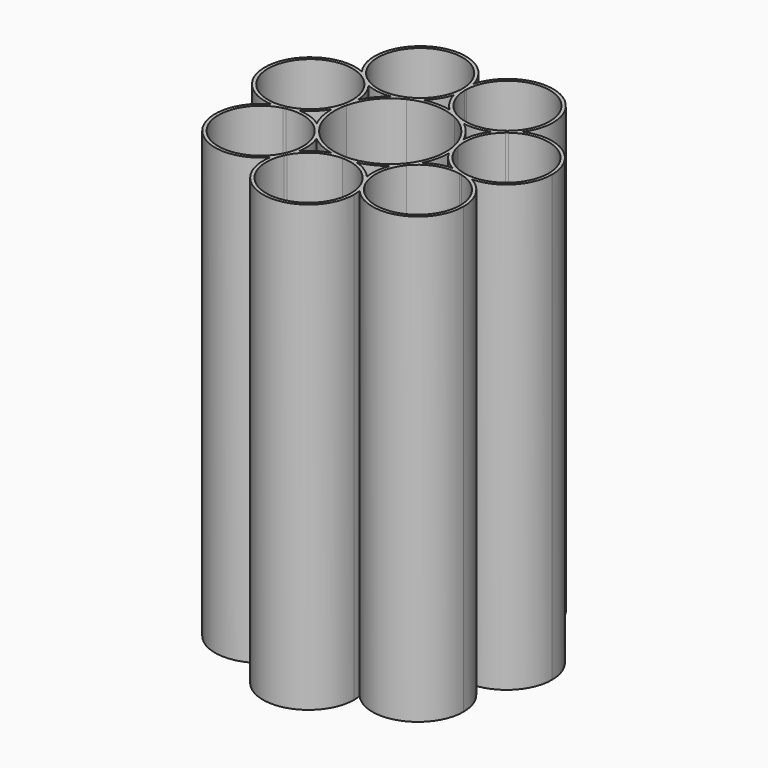
from build123d import *

# Parameters (mm, degrees)
F1_DEPTH = 100
F2_DEPTH = 1.5


with BuildPart() as f1:
    # F0 (on Top) → F1 (new body)
    with BuildSketch(Plane.XY):
        with BuildLine():
            ThreePointArc((48.1206952739, 11.3566633912), (48.7132972202, 9.4977687695), (48.9136480771, 7.5570148398))
            ThreePointArc((48.9136480771, 7.5570148398), (37.405752333, -1.7283690877), (30.7624155128, 11.4820849178))
            ThreePointArc((30.7624155128, 11.4820849178), (30.1118696666, 10.4093871837), (29.3351499151, 9.4241984938))
            ThreePointArc((29.3351499151, 9.4241984938), (38.476126387, -2.6500196502), (49.6636480771, 7.5570148398))
            ThreePointArc((49.6636480771, 7.5570148398), (49.6271899841, 8.4207634811), (49.5180750595, 9.2783676097))
            ThreePointArc((49.5180750595, 9.2783676097), (48.755672541, 10.2746771633), (48.1206952739, 11.3566633912))
        make_face()
        with BuildLine():
            ThreePointArc((47.8763467124, 11.8735796555), (48.0024107115, 11.6169602101), (48.1206952739, 11.3566633912))
            ThreePointArc((48.1206952739, 11.3566633912), (48.755672541, 10.2746771633), (49.5180750595, 9.2783676097))
            ThreePointArc((49.5180750595, 9.2783676097), (49.2321003695, 10.4998866655), (48.7990402105, 11.6773199866))
            ThreePointArc((48.7990402105, 11.6773199866), (48.6729762114, 11.933939432), (48.5546916491, 12.1942362509))
            ThreePointArc((48.5546916491, 12.1942362509), (47.919714382, 13.2762224787), (47.1573118635, 14.2725320324))
            ThreePointArc((47.1573118635, 14.2725320324), (47.4432865534, 13.0510129766), (47.8763467124, 11.8735796555))
        make_face()
        with BuildLine():
            ThreePointArc((29.3351499151, 9.4241984938), (30.1118696666, 10.4093871837), (30.7624155128, 11.4820849178))
            ThreePointArc((30.7624155128, 11.4820849178), (30.8844490564, 11.7406453283), (31.0142080859, 11.9954163351))
            ThreePointArc((31.0142080859, 11.9954163351), (31.464237132, 13.1664689319), (31.7678331121, 14.3837280695))
            ThreePointArc((31.7678331121, 14.3837280695), (30.9911133606, 13.3985393796), (30.3405675144, 12.3258416454))
            ThreePointArc((30.3405675144, 12.3258416454), (30.2185339708, 12.0672812349), (30.0887749413, 11.8125102282))
            ThreePointArc((30.0887749413, 11.8125102282), (29.6387458952, 10.6414576313), (29.3351499151, 9.4241984938))
        make_face()
        with BuildLine():
            ThreePointArc((39.4822879755, 17.0567668662), (44.4048695418, 15.6401892342), (47.8763467124, 11.8735796555))
            ThreePointArc((47.8763467124, 11.8735796555), (47.4432865534, 13.0510129766), (47.1573118635, 14.2725320324))
            ThreePointArc((47.1573118635, 14.2725320324), (44.9982610803, 16.1520481501), (42.4036526816, 17.3612166158))
            ThreePointArc((42.4036526816, 17.3612166158), (40.9514324879, 17.1277926143), (39.4822879755, 17.0567668662))
        make_face()
        with BuildLine():
            ThreePointArc((48.7990402105, 11.6773199866), (49.2321003695, 10.4998866655), (49.5180750595, 9.2783676097))
            ThreePointArc((49.5180750595, 9.2783676097), (60.8457272798, 6.3908890767), (67.5117388458, 15.9938848023))
            ThreePointArc((67.5117388458, 15.9938848023), (66.0890556448, 21.20358519), (62.215938235, 24.9670898268))
            ThreePointArc((62.215938235, 24.9670898268), (60.9616418645, 24.9922083817), (59.7198091175, 25.1703705424))
            ThreePointArc((59.7198091175, 25.1703705424), (64.7983716344, 21.7774102159), (66.7617388458, 15.9938848023))
            ThreePointArc((66.7617388458, 15.9938848023), (59.4814643879, 6.7568496439), (48.7990402105, 11.6773199866))
        make_face()
        with BuildLine():
            ThreePointArc((31.7678331121, 14.3837280695), (31.464237132, 13.1664689319), (31.0142080859, 11.9954163351))
            ThreePointArc((31.0142080859, 11.9954163351), (34.5397507817, 15.7114691534), (39.4822879755, 17.0567668662))
            ThreePointArc((39.4822879755, 17.0567668662), (38.0143233536, 17.149014592), (36.5656279622, 17.40339902))
            ThreePointArc((36.5656279622, 17.40339902), (33.9538177836, 16.2318493146), (31.7678331121, 14.3837280695))
        make_face()
        with BuildLine():
            ThreePointArc((16.8653170922, 25.294768849), (13.6295963948, 9.9182097392), (29.3351499151, 9.4241984938))
            ThreePointArc((29.3351499151, 9.4241984938), (29.6387458952, 10.6414576313), (30.0887749413, 11.8125102282))
            ThreePointArc((30.0887749413, 11.8125102282), (14.2193333623, 10.3815781771), (19.3641230306, 25.4619588697))
            ThreePointArc((19.3641230306, 25.4619588697), (18.1198454701, 25.3017599953), (16.8653170922, 25.294768849))
        make_face()
        with BuildLine():
            ThreePointArc((36.5656279622, 17.40339902), (38.0143233536, 17.149014592), (39.4822879755, 17.0567668662))
            ThreePointArc((39.4822879755, 17.0567668662), (40.9514324879, 17.1277926143), (42.4036526816, 17.3612166158))
            ThreePointArc((42.4036526816, 17.3612166158), (40.9617908418, 17.6894259043), (39.4877071959, 17.8067472874))
            ThreePointArc((39.4877071959, 17.8067472874), (38.0120820394, 17.7107389173), (36.5656279622, 17.40339902))
        make_face()
        with BuildLine():
            ThreePointArc((47.7878142081, 19.9063331353), (47.0753316403, 17.1338884178), (47.1573118635, 14.2725320324))
            ThreePointArc((47.1573118635, 14.2725320324), (47.919714382, 13.2762224787), (48.5546916491, 12.1942362509))
            ThreePointArc((48.5546916491, 12.1942362509), (47.8475044956, 17.2675376586), (49.8773300395, 21.9705483013))
            ThreePointArc((49.8773300395, 21.9705483013), (48.8899468368, 20.8803627751), (47.7878142081, 19.9063331353))
        make_face()
        with BuildLine():
            ThreePointArc((30.3405675144, 12.3258416454), (30.9911133606, 13.3985393796), (31.7678331121, 14.3837280695))
            ThreePointArc((31.7678331121, 14.3837280695), (31.8963694401, 15.3133900333), (31.9393349501, 16.2509117234))
            ThreePointArc((31.9393349501, 16.2509117234), (31.7575914431, 18.1725545596), (31.2188059374, 20.0260518137))
            ThreePointArc((31.2188059374, 20.0260518137), (30.1308632886, 21.0159057298), (29.1593365515, 22.1202452524))
            ThreePointArc((29.1593365515, 22.1202452524), (30.6675033383, 19.3561480096), (31.1893349501, 16.2509117234))
            ThreePointArc((31.1893349501, 16.2509117234), (30.9747188775, 14.2430159793), (30.3405675144, 12.3258416454))
        make_face()
        with BuildLine():
            ThreePointArc((19.2024519144, 26.1946490876), (18.0062976057, 25.8163566122), (16.8653170922, 25.294768849))
            ThreePointArc((16.8653170922, 25.294768849), (18.1198454701, 25.3017599953), (19.3641230306, 25.4619588697))
            ThreePointArc((19.3641230306, 25.4619588697), (19.6423603695, 25.5277589824), (19.922451795, 25.5851564126))
            ThreePointArc((19.922451795, 25.5851564126), (21.1186061037, 25.9634488879), (22.2595866172, 26.4850366512))
            ThreePointArc((22.2595866172, 26.4850366512), (21.0050582393, 26.4780455049), (19.7607806788, 26.3178466305))
            ThreePointArc((19.7607806788, 26.3178466305), (19.4825433399, 26.2520465177), (19.2024519144, 26.1946490876))
        make_face()
        with BuildLine():
            ThreePointArc((21.4986150447, 44.9392154972), (7.4592981841, 37.8818760143), (16.8653170922, 25.294768849))
            ThreePointArc((16.8653170922, 25.294768849), (18.0062976057, 25.8163566122), (19.2024519144, 26.1946490876))
            ThreePointArc((19.2024519144, 26.1946490876), (8.1892692018, 37.7097065822), (23.1873094858, 43.0898116188))
            ThreePointArc((23.1873094858, 43.0898116188), (22.2862665927, 43.9627446242), (21.4986150447, 44.9392154972))
        make_face()
        with BuildLine():
            ThreePointArc((31.2188059374, 20.0260518137), (33.7429593868, 18.4104328977), (36.5656279622, 17.40339902))
            ThreePointArc((36.5656279622, 17.40339902), (38.0120820394, 17.7107389173), (39.4877071959, 17.8067472874))
            ThreePointArc((39.4877071959, 17.8067472874), (34.0732460725, 19.0837906816), (29.7490735348, 22.5836136702))
            ThreePointArc((29.7490735348, 22.5836136702), (30.5764241251, 21.3579799622), (31.2188059374, 20.0260518137))
        make_face()
        with BuildLine():
            ThreePointArc((39.4877071959, 17.8067472874), (40.9617908418, 17.6894259043), (42.4036526816, 17.3612166158))
            ThreePointArc((42.4036526816, 17.3612166158), (45.2405783478, 18.3273573313), (47.7878142081, 19.9063331353))
            ThreePointArc((47.7878142081, 19.9063331353), (48.4493754616, 21.2288395857), (49.2943501781, 22.4423898862))
            ThreePointArc((49.2943501781, 22.4423898862), (44.9200562534, 19.005417496), (39.4877071959, 17.8067472874))
        make_face()
        with BuildLine():
            ThreePointArc((49.2943501781, 22.4423898862), (48.4493754616, 21.2288395857), (47.7878142081, 19.9063331353))
            ThreePointArc((47.7878142081, 19.9063331353), (48.8899468368, 20.8803627751), (49.8773300395, 21.9705483013))
            ThreePointArc((49.8773300395, 21.9705483013), (50.737796422, 23.1634554911), (51.4607426152, 24.4443843575))
            ThreePointArc((51.4607426152, 24.4443843575), (50.3051519569, 23.5217263825), (49.2943501781, 22.4423898862))
        make_face()
        with BuildLine():
            ThreePointArc((59.7198091175, 25.1703705424), (60.9616418645, 24.9922083817), (62.215938235, 24.9670898268))
            ThreePointArc((62.215938235, 24.9670898268), (61.082613878, 25.505110485), (59.8920508463, 25.900648087))
            ThreePointArc((59.8920508463, 25.900648087), (59.612818067, 25.9620868909), (59.3355606009, 26.0319007082))
            ThreePointArc((59.3355606009, 26.0319007082), (58.0937278539, 26.210062869), (56.8394314834, 26.2351814239))
            ThreePointArc((56.8394314834, 26.2351814239), (57.9727558404, 25.6971607656), (59.1633188721, 25.3016231636))
            ThreePointArc((59.1633188721, 25.3016231636), (59.4425516513, 25.2401843598), (59.7198091175, 25.1703705424))
        make_face()
        with BuildLine():
            ThreePointArc((59.8920508463, 25.900648087), (61.082613878, 25.505110485), (62.215938235, 24.9670898268))
            ThreePointArc((62.215938235, 24.9670898268), (69.1892765667, 28.1114205638), (72.0436308726, 35.2083864484))
            ThreePointArc((72.0436308726, 35.2083864484), (67.4863642116, 43.732193528), (57.8669894813, 44.6764373241))
            ThreePointArc((57.8669894813, 44.6764373241), (57.0653100087, 43.711450096), (56.1517471691, 42.8516284488))
            ThreePointArc((56.1517471691, 42.8516284488), (66.0745247522, 43.6891852074), (71.2936308726, 35.2083864484))
            ThreePointArc((71.2936308726, 35.2083864484), (67.8013338342, 27.849208157), (59.8920508463, 25.900648087))
        make_face()
        with BuildLine():
            ThreePointArc((23.6593494729, 43.6730360661), (22.6177984932, 44.372365662), (21.4986150447, 44.9392154972))
            ThreePointArc((21.4986150447, 44.9392154972), (22.2862665927, 43.9627446242), (23.1873094858, 43.0898116188))
            ThreePointArc((23.1873094858, 43.0898116188), (23.4122322289, 42.913302607), (23.6317414941, 42.7301050249))
            ThreePointArc((23.6317414941, 42.7301050249), (24.6732924738, 42.030775429), (25.7924759223, 41.4639255938))
            ThreePointArc((25.7924759223, 41.4639255938), (25.0048243743, 42.4403964668), (24.1037814812, 43.3133294722))
            ThreePointArc((24.1037814812, 43.3133294722), (23.8788587381, 43.489838484), (23.6593494729, 43.6730360661))
        make_face()
        with BuildLine():
            ThreePointArc((39.7460759123, 53.5648694386), (25.4750548344, 60.1410701567), (21.4986150447, 44.9392154972))
            ThreePointArc((21.4986150447, 44.9392154972), (22.6177984932, 44.372365662), (23.6593494729, 43.6730360661))
            ThreePointArc((23.6593494729, 43.6730360661), (25.7955768373, 59.4630099487), (39.3530374989, 51.0915105026))
            ThreePointArc((39.3530374989, 51.0915105026), (39.4737329496, 52.34023903), (39.7460759123, 53.5648694386))
        make_face()
        with BuildLine():
            ThreePointArc((29.1593365515, 22.1202452524), (30.1308632886, 21.0159057298), (31.2188059374, 20.0260518137))
            ThreePointArc((31.2188059374, 20.0260518137), (30.5764241251, 21.3579799622), (29.7490735348, 22.5836136702))
            ThreePointArc((29.7490735348, 22.5836136702), (28.7539739464, 23.6774436092), (27.6118365935, 24.6167036336))
            ThreePointArc((27.6118365935, 24.6167036336), (28.3161976905, 23.3254617924), (29.1593365515, 22.1202452524))
        make_face()
        with BuildLine():
            ThreePointArc((51.4607426152, 24.4443843575), (50.737796422, 23.1634554911), (49.8773300395, 21.9705483013))
            ThreePointArc((49.8773300395, 21.9705483013), (54.054034403, 24.935955715), (59.1633188721, 25.3016231636))
            ThreePointArc((59.1633188721, 25.3016231636), (57.9727558404, 25.6971607656), (56.8394314834, 26.2351814239))
            ThreePointArc((56.8394314834, 26.2351814239), (54.0238204657, 25.7190266811), (51.4607426152, 24.4443843575))
        make_face()
        with BuildLine():
            ThreePointArc((52.0780229629, 30.3064210056), (51.3615727292, 26.1353354269), (49.2943501781, 22.4423898862))
            ThreePointArc((49.2943501781, 22.4423898862), (50.3051519569, 23.5217263825), (51.4607426152, 24.4443843575))
            ThreePointArc((51.4607426152, 24.4443843575), (52.4741776089, 27.26476104), (52.8278601971, 30.24074554))
            ThreePointArc((52.8278601971, 30.24074554), (52.2063596702, 31.5825443542), (51.7844009488, 32.9998085498))
            ThreePointArc((51.7844009488, 32.9998085498), (52.0044006496, 31.6610935076), (52.0780229629, 30.3064210056))
        make_face()
        with BuildLine():
            ThreePointArc((22.2595866172, 26.4850366512), (21.1186061037, 25.9634488879), (19.922451795, 25.5851564126))
            ThreePointArc((19.922451795, 25.5851564126), (25.0259188828, 25.145697143), (29.1593365515, 22.1202452524))
            ThreePointArc((29.1593365515, 22.1202452524), (28.3161976905, 23.3254617924), (27.6118365935, 24.6167036336))
            ThreePointArc((27.6118365935, 24.6167036336), (25.0674451398, 25.9282497637), (22.2595866172, 26.4850366512))
        make_face()
        with BuildLine():
            ThreePointArc((40.1033328511, 51.0860892748), (40.0006943318, 52.3364314925), (39.7460759123, 53.5648694386))
            ThreePointArc((39.7460759123, 53.5648694386), (39.4737329496, 52.34023903), (39.3530374989, 51.0915105026))
            ThreePointArc((39.3530374989, 51.0915105026), (39.3549010101, 50.9828860122), (39.3555222076, 50.8742473143))
            ThreePointArc((39.3555222076, 50.8742473143), (39.3538681077, 50.6969758782), (39.3489063841, 50.5197661737))
            ThreePointArc((39.3489063841, 50.5197661737), (39.4515449033, 49.269423956), (39.7061633229, 48.0409860099))
            ThreePointArc((39.7061633229, 48.0409860099), (39.9785062855, 49.2656164185), (40.0992017363, 50.5143449459))
            ThreePointArc((40.0992017363, 50.5143449459), (40.0969650022, 50.8002481964), (40.1033328511, 51.0860892748))
        make_face()
        with BuildLine():
            ThreePointArc((59.8467170275, 50.7316081342), (51.0273512521, 60.8812773759), (39.7460759123, 53.5648694386))
            ThreePointArc((39.7460759123, 53.5648694386), (40.0006943318, 52.3364314925), (40.1033328511, 51.0860892748))
            ThreePointArc((40.1033328511, 51.0860892748), (49.7739884636, 60.2299540343), (59.0967170275, 50.7316081342))
            ThreePointArc((59.0967170275, 50.7316081342), (58.2024981574, 46.7078622248), (55.6881841552, 43.4416130565))
            ThreePointArc((55.6881841552, 43.4416130565), (56.7397318136, 44.1258190555), (57.8669894813, 44.6764373241))
            ThreePointArc((57.8669894813, 44.6764373241), (59.3392216503, 47.5463132225), (59.8467170275, 50.7316081342))
        make_face()
        with BuildLine():
            ThreePointArc((26.68186832, 33.3480809845), (24.2054297809, 28.8641370859), (19.7607806788, 26.3178466305))
            ThreePointArc((19.7607806788, 26.3178466305), (21.0050582393, 26.4780455049), (22.2595866172, 26.4850366512))
            ThreePointArc((22.2595866172, 26.4850366512), (24.5724133385, 28.1717238416), (26.3286201104, 30.4322146944))
            ThreePointArc((26.3286201104, 30.4322146944), (26.4241979206, 31.8999663481), (26.68186832, 33.3480809845))
        make_face()
        with BuildLine():
            ThreePointArc((27.6118365935, 24.6167036336), (28.7539739464, 23.6774436092), (29.7490735348, 22.5836136702))
            ThreePointArc((29.7490735348, 22.5836136702), (27.3716449829, 27.613033434), (27.4118393617, 33.1759116542))
            ThreePointArc((27.4118393617, 33.1759116542), (26.9694449908, 31.7648927136), (26.3286201104, 30.4322146944))
            ThreePointArc((26.3286201104, 30.4322146944), (26.6392623122, 27.4514301433), (27.6118365935, 24.6167036336))
        make_face()
        with BuildLine():
            ThreePointArc((56.8394314834, 26.2351814239), (58.0937278539, 26.210062869), (59.3355606009, 26.0319007082))
            ThreePointArc((59.3355606009, 26.0319007082), (54.9281698401, 28.64215124), (52.5167835917, 33.1614119671))
            ThreePointArc((52.5167835917, 33.1614119671), (52.7499833016, 31.7423739415), (52.8280229629, 30.3064210056))
            ThreePointArc((52.8280229629, 30.3064210056), (52.8279822714, 30.2735831719), (52.8278601971, 30.24074554))
            ThreePointArc((52.8278601971, 30.24074554), (54.5512191456, 27.9551132302), (56.8394314834, 26.2351814239))
        make_face()
        with BuildLine():
            ThreePointArc((56.1517471691, 42.8516284488), (57.0653100087, 43.711450096), (57.8669894813, 44.6764373241))
            ThreePointArc((57.8669894813, 44.6764373241), (56.7397318136, 44.1258190555), (55.6881841552, 43.4416130565))
            ThreePointArc((55.6881841552, 43.4416130565), (55.4660505739, 43.2616065464), (55.238600731, 43.0883661338))
            ThreePointArc((55.238600731, 43.0883661338), (54.3250378913, 42.2285444866), (53.5233584188, 41.2635572585))
            ThreePointArc((53.5233584188, 41.2635572585), (54.6506160864, 41.8141755271), (55.7021637449, 42.4983815261))
            ThreePointArc((55.7021637449, 42.4983815261), (55.9242973262, 42.6783880362), (56.1517471691, 42.8516284488))
        make_face()
        with BuildLine():
            ThreePointArc((25.7924759223, 41.4639255938), (24.6732924738, 42.030775429), (23.6317414941, 42.7301050249))
            ThreePointArc((23.6317414941, 42.7301050249), (26.0701979054, 39.4903555662), (26.9355687593, 35.5288937767))
            ThreePointArc((26.9355687593, 35.5288937767), (26.8719305007, 34.4311337452), (26.68186832, 33.3480809845))
            ThreePointArc((26.68186832, 33.3480809845), (27.0984560706, 34.7587136939), (27.6688276266, 36.1144814773))
            ThreePointArc((27.6688276266, 36.1144814773), (27.1078335586, 38.9215024564), (25.7924759223, 41.4639255938))
        make_face()
        with BuildLine():
            ThreePointArc((33.9154678115, 42.2854847903), (28.8657450324, 41.4259489943), (24.1037814812, 43.3133294722))
            ThreePointArc((24.1037814812, 43.3133294722), (25.0048243743, 42.4403964668), (25.7924759223, 41.4639255938))
            ThreePointArc((25.7924759223, 41.4639255938), (28.5532049431, 40.7073171118), (31.4155048698, 40.7436523617))
            ThreePointArc((31.4155048698, 40.7436523617), (32.6226312153, 41.5840548726), (33.9154678115, 42.2854847903))
        make_face()
        with BuildLine():
            ThreePointArc((27.6688276266, 36.1144814773), (27.0984560706, 34.7587136939), (26.68186832, 33.3480809845))
            ThreePointArc((26.68186832, 33.3480809845), (26.4241979206, 31.8999663481), (26.3286201104, 30.4322146944))
            ThreePointArc((26.3286201104, 30.4322146944), (26.9694449908, 31.7648927136), (27.4118393617, 33.1759116542))
            ThreePointArc((27.4118393617, 33.1759116542), (27.6169064336, 34.3444685309), (27.6855687593, 35.5288937767))
            ThreePointArc((27.6855687593, 35.5288937767), (27.6813826214, 35.821807254), (27.6688276266, 36.1144814773))
        make_face()
        with BuildLine():
            ThreePointArc((27.6855687593, 35.5288937767), (27.6169064336, 34.3444685309), (27.4118393617, 33.1759116542))
            ThreePointArc((27.4118393617, 33.1759116542), (29.8616956216, 38.1704519693), (34.2359896665, 41.6074245124))
            ThreePointArc((34.2359896665, 41.6074245124), (32.8569822677, 41.0735464461), (31.4155048698, 40.7436523617))
            ThreePointArc((31.4155048698, 40.7436523617), (29.2787159102, 38.6422937394), (27.6688276266, 36.1144814773))
            ThreePointArc((27.6688276266, 36.1144814773), (27.6813826214, 35.821807254), (27.6855687593, 35.5288937767))
        make_face()
        with BuildLine():
            ThreePointArc((51.7844009488, 32.9998085498), (52.2063596702, 31.5825443542), (52.8278601971, 30.24074554))
            ThreePointArc((52.8278601971, 30.24074554), (52.8279822714, 30.2735831719), (52.8280229629, 30.3064210056))
            ThreePointArc((52.8280229629, 30.3064210056), (52.7499833016, 31.7423739415), (52.5167835917, 33.1614119671))
            ThreePointArc((52.5167835917, 33.1614119671), (52.1206232128, 34.5779171099), (51.5699022873, 35.9417852589))
            ThreePointArc((51.5699022873, 35.9417852589), (51.5707663403, 34.4630403849), (51.7844009488, 32.9998085498))
        make_face()
        with BuildLine():
            ThreePointArc((45.0828000959, 41.5290512105), (49.4069725, 38.0292282022), (51.7844009488, 32.9998085498))
            ThreePointArc((51.7844009488, 32.9998085498), (51.5707663403, 34.4630403849), (51.5699022873, 35.9417852589))
            ThreePointArc((51.5699022873, 35.9417852589), (49.9967093879, 38.4925967413), (47.8905085013, 40.6246129099))
            ThreePointArc((47.8905085013, 40.6246129099), (46.4539487673, 40.9753020883), (45.0828000959, 41.5290512105))
        make_face()
        with BuildLine():
            ThreePointArc((51.5699022873, 35.9417852589), (52.1206232128, 34.5779171099), (52.5167835917, 33.1614119671))
            ThreePointArc((52.5167835917, 33.1614119671), (52.8024673174, 38.2757921802), (55.7021637449, 42.4983815261))
            ThreePointArc((55.7021637449, 42.4983815261), (54.6506160864, 41.8141755271), (53.5233584188, 41.2635572585))
            ThreePointArc((53.5233584188, 41.2635572585), (52.171399691, 38.7404067043), (51.5699022873, 35.9417852589))
        make_face()
        with BuildLine():
            ThreePointArc((39.7061633229, 48.0409860099), (39.4515449033, 49.269423956), (39.3489063841, 50.5197661737))
            ThreePointArc((39.3489063841, 50.5197661737), (37.7848370903, 45.6420426651), (33.9154678115, 42.2854847903))
            ThreePointArc((33.9154678115, 42.2854847903), (35.2780829825, 42.8392984152), (36.6936856513, 43.238671323))
            ThreePointArc((36.6936856513, 43.238671323), (38.5385289443, 45.4274231009), (39.7061633229, 48.0409860099))
        make_face()
        with BuildLine():
            ThreePointArc((45.4130863949, 42.2024091841), (41.5926238575, 45.6145296195), (40.0992017363, 50.5143449459))
            ThreePointArc((40.0992017363, 50.5143449459), (39.9785062855, 49.2656164185), (39.7061633229, 48.0409860099))
            ThreePointArc((39.7061633229, 48.0409860099), (40.8359093819, 45.4108234744), (42.6489322384, 43.1956419371))
            ThreePointArc((42.6489322384, 43.1956419371), (44.0586161482, 42.7758550227), (45.4130863949, 42.2024091841))
        make_face()
        with BuildLine():
            ThreePointArc((36.6936856513, 43.238671323), (35.2780829825, 42.8392984152), (33.9154678115, 42.2854847903))
            ThreePointArc((33.9154678115, 42.2854847903), (32.6226312153, 41.5840548726), (31.4155048698, 40.7436523617))
            ThreePointArc((31.4155048698, 40.7436523617), (32.8569822677, 41.0735464461), (34.2359896665, 41.6074245124))
            ThreePointArc((34.2359896665, 41.6074245124), (35.5238254256, 42.3341747953), (36.6936856513, 43.238671323))
        make_face()
        with BuildLine():
            ThreePointArc((36.6936856513, 43.238671323), (35.5238254256, 42.3341747953), (34.2359896665, 41.6074245124))
            ThreePointArc((34.2359896665, 41.6074245124), (39.6683389786, 42.806094722), (45.0828000959, 41.5290512105))
            ThreePointArc((45.0828000959, 41.5290512105), (43.8056003177, 42.2743350954), (42.6489322384, 43.1956419371))
            ThreePointArc((42.6489322384, 43.1956419371), (39.6737577864, 43.5560751461), (36.6936856513, 43.238671323))
        make_face()
        with BuildLine():
            ThreePointArc((42.6489322384, 43.1956419371), (43.8056003177, 42.2743350954), (45.0828000959, 41.5290512105))
            ThreePointArc((45.0828000959, 41.5290512105), (46.4539487673, 40.9753020883), (47.8905085013, 40.6246129099))
            ThreePointArc((47.8905085013, 40.6246129099), (46.6956521847, 41.4823708203), (45.4130863949, 42.2024091841))
            ThreePointArc((45.4130863949, 42.2024091841), (44.0586161482, 42.7758550227), (42.6489322384, 43.1956419371))
        make_face()
        with BuildLine():
            ThreePointArc((53.5233584188, 41.2635572585), (54.3250378913, 42.2285444866), (55.238600731, 43.0883661338))
            ThreePointArc((55.238600731, 43.0883661338), (50.4498614665, 41.2699938657), (45.4130863949, 42.2024091841))
            ThreePointArc((45.4130863949, 42.2024091841), (46.6956521847, 41.4823708203), (47.8905085013, 40.6246129099))
            ThreePointArc((47.8905085013, 40.6246129099), (50.7519845278, 40.5469207555), (53.5233584188, 41.2635572585))
        make_face()
    extrude(amount=F1_DEPTH)

    # F0 (on Top) → F2 (join)
    with BuildSketch(Plane.XY):
        with BuildLine():
            ThreePointArc((30.7624155128, 11.4820849178), (37.405752333, -1.7283690877), (48.9136480771, 7.5570148398))
            ThreePointArc((48.9136480771, 7.5570148398), (48.7132972202, 9.4977687695), (48.1206952739, 11.3566633912))
            ThreePointArc((48.1206952739, 11.3566633912), (47.9949160034, 11.613417429), (47.8763467124, 11.8735796555))
            ThreePointArc((47.8763467124, 11.8735796555), (44.4048695418, 15.6401892342), (39.4822879755, 17.0567668662))
            ThreePointArc((39.4822879755, 17.0567668662), (34.5397507817, 15.7114691534), (31.0142080859, 11.9954163351))
            ThreePointArc((31.0142080859, 11.9954163351), (30.8918917882, 11.7369946174), (30.7624155128, 11.4820849178))
        make_face()
        with BuildLine():
            ThreePointArc((39.4822879755, 17.0567668662), (44.4048695418, 15.6401892342), (47.8763467124, 11.8735796555))
            ThreePointArc((47.8763467124, 11.8735796555), (47.4432865534, 13.0510129766), (47.1573118635, 14.2725320324))
            ThreePointArc((47.1573118635, 14.2725320324), (44.9982610803, 16.1520481501), (42.4036526816, 17.3612166158))
            ThreePointArc((42.4036526816, 17.3612166158), (40.9514324879, 17.1277926143), (39.4822879755, 17.0567668662))
        make_face()
        with BuildLine():
            ThreePointArc((48.5546916491, 12.1942362509), (48.6804709195, 11.937482213), (48.7990402105, 11.6773199866))
            ThreePointArc((48.7990402105, 11.6773199866), (59.4814643879, 6.7568496439), (66.7617388458, 15.9938848023))
            ThreePointArc((66.7617388458, 15.9938848023), (64.7983716344, 21.7774102159), (59.7198091175, 25.1703705424))
            ThreePointArc((59.7198091175, 25.1703705424), (59.440648635, 25.2321158732), (59.1633188721, 25.3016231636))
            ThreePointArc((59.1633188721, 25.3016231636), (54.054034403, 24.935955715), (49.8773300395, 21.9705483013))
            ThreePointArc((49.8773300395, 21.9705483013), (47.8475044956, 17.2675376586), (48.5546916491, 12.1942362509))
        make_face()
        with BuildLine():
            ThreePointArc((19.3641230306, 25.4619588697), (14.2193333623, 10.3815781771), (30.0887749413, 11.8125102282))
            ThreePointArc((30.0887749413, 11.8125102282), (30.211091239, 12.0709319458), (30.3405675144, 12.3258416454))
            ThreePointArc((30.3405675144, 12.3258416454), (30.9747188775, 14.2430159793), (31.1893349501, 16.2509117234))
            ThreePointArc((31.1893349501, 16.2509117234), (30.6675033383, 19.3561480096), (29.1593365515, 22.1202452524))
            ThreePointArc((29.1593365515, 22.1202452524), (25.0259188828, 25.145697143), (19.922451795, 25.5851564126))
            ThreePointArc((19.922451795, 25.5851564126), (19.6441465962, 25.5196638394), (19.3641230306, 25.4619588697))
        make_face()
        with BuildLine():
            ThreePointArc((23.1873094858, 43.0898116188), (8.1892692018, 37.7097065822), (19.2024519144, 26.1946490876))
            ThreePointArc((19.2024519144, 26.1946490876), (19.4807571132, 26.2601416608), (19.7607806788, 26.3178466305))
            ThreePointArc((19.7607806788, 26.3178466305), (24.2054297809, 28.8641370859), (26.68186832, 33.3480809845))
            ThreePointArc((26.68186832, 33.3480809845), (26.8719305007, 34.4311337452), (26.9355687593, 35.5288937767))
            ThreePointArc((26.9355687593, 35.5288937767), (26.0701979054, 39.4903555662), (23.6317414941, 42.7301050249))
            ThreePointArc((23.6317414941, 42.7301050249), (23.4070168853, 42.9068588395), (23.1873094858, 43.0898116188))
        make_face()
        with BuildLine():
            ThreePointArc((29.7490735348, 22.5836136702), (34.0732460725, 19.0837906816), (39.4877071959, 17.8067472874))
            ThreePointArc((39.4877071959, 17.8067472874), (44.9200562534, 19.005417496), (49.2943501781, 22.4423898862))
            ThreePointArc((49.2943501781, 22.4423898862), (51.3615727292, 26.1353354269), (52.0780229629, 30.3064210056))
            ThreePointArc((52.0780229629, 30.3064210056), (52.0044006496, 31.6610935076), (51.7844009488, 32.9998085498))
            ThreePointArc((51.7844009488, 32.9998085498), (49.4069725, 38.0292282022), (45.0828000959, 41.5290512105))
            ThreePointArc((45.0828000959, 41.5290512105), (39.6683389786, 42.806094722), (34.2359896665, 41.6074245124))
            ThreePointArc((34.2359896665, 41.6074245124), (29.8616956216, 38.1704519693), (27.4118393617, 33.1759116542))
            ThreePointArc((27.4118393617, 33.1759116542), (27.3716449829, 27.613033434), (29.7490735348, 22.5836136702))
        make_face()
        with BuildLine():
            ThreePointArc((59.3355606009, 26.0319007082), (59.6147210834, 25.9701553775), (59.8920508463, 25.900648087))
            ThreePointArc((59.8920508463, 25.900648087), (67.8013338342, 27.849208157), (71.2936308726, 35.2083864484))
            ThreePointArc((71.2936308726, 35.2083864484), (66.0745247522, 43.6891852074), (56.1517471691, 42.8516284488))
            ThreePointArc((56.1517471691, 42.8516284488), (55.9294190118, 42.671869579), (55.7021637449, 42.4983815261))
            ThreePointArc((55.7021637449, 42.4983815261), (52.8024673174, 38.2757921802), (52.5167835917, 33.1614119671))
            ThreePointArc((52.5167835917, 33.1614119671), (54.9281698401, 28.64215124), (59.3355606009, 26.0319007082))
        make_face()
        with BuildLine():
            ThreePointArc((39.3530374989, 51.0915105026), (25.7955768373, 59.4630099487), (23.6593494729, 43.6730360661))
            ThreePointArc((23.6593494729, 43.6730360661), (23.8840740817, 43.4962822514), (24.1037814812, 43.3133294722))
            ThreePointArc((24.1037814812, 43.3133294722), (28.8657450324, 41.4259489943), (33.9154678115, 42.2854847903))
            ThreePointArc((33.9154678115, 42.2854847903), (37.7848370903, 45.6420426651), (39.3489063841, 50.5197661737))
            ThreePointArc((39.3489063841, 50.5197661737), (39.3469845792, 50.8056671487), (39.3530374989, 51.0915105026))
        make_face()
        with BuildLine():
            ThreePointArc((59.0967170275, 50.7316081342), (49.7739884636, 60.2299540343), (40.1033328511, 51.0860892748))
            ThreePointArc((40.1033328511, 51.0860892748), (40.1049748539, 50.9801739511), (40.1055222076, 50.8742473143))
            ThreePointArc((40.1055222076, 50.8742473143), (40.103941968, 50.6942683828), (40.0992017363, 50.5143449459))
            ThreePointArc((40.0992017363, 50.5143449459), (41.5926238575, 45.6145296195), (45.4130863949, 42.2024091841))
            ThreePointArc((45.4130863949, 42.2024091841), (50.4498614665, 41.2699938657), (55.238600731, 43.0883661338))
            ThreePointArc((55.238600731, 43.0883661338), (55.4609288883, 43.2681250036), (55.6881841552, 43.4416130565))
            ThreePointArc((55.6881841552, 43.4416130565), (58.2024981574, 46.7078622248), (59.0967170275, 50.7316081342))
        make_face()
    extrude(amount=F2_DEPTH)


solid = f1.part
